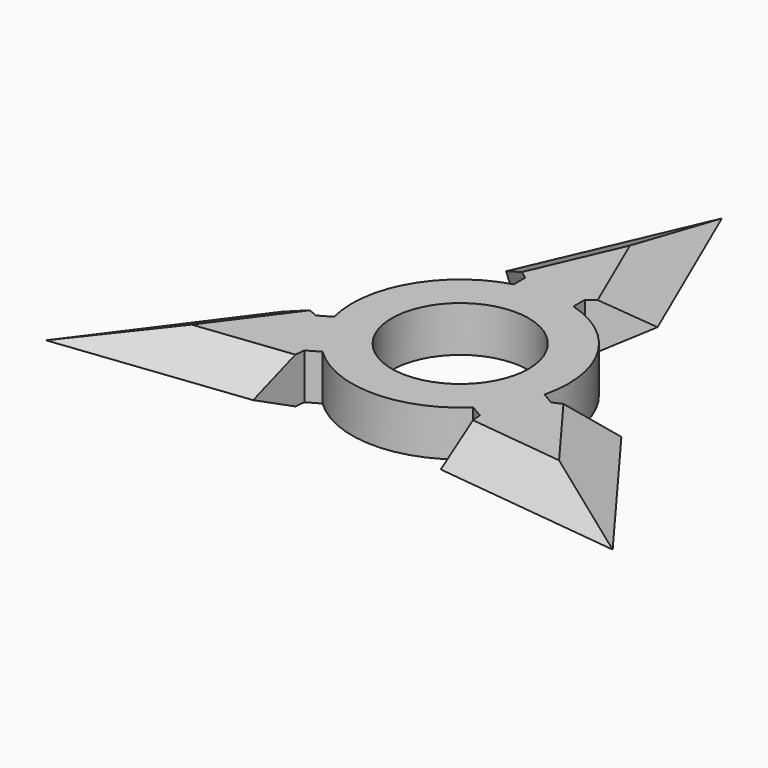
from build123d import *

# Parameters (mm, degrees)
F0_R            = 15.08125
F0_R_2          = 9.525
F1_DEPTH        = 6.35
F3_DEPTH        = 6.35
F3_COPIES_COUNT = 3
F4_SIZE2        = 3.175
F4_SIZE         = 6.35
F4_2_SIZE2      = 3.17499
F4_2_SIZE       = 6.34999


# Not quite as in the source:
# - a fillet or chamfer is up to 0.001 mm smaller than in the source, because OpenCascade refuses the exact size
# - a pattern or mirror of a feature is missing from the dataset's text; its kind, count and spacing are read off the source's solid


with BuildPart() as f1:
    # F0 (on Top) → F1 (new body)
    with BuildSketch(Plane.XY):
        Circle(F0_R)
        Circle(F0_R_2, mode=Mode.SUBTRACT)
    extrude(amount=F1_DEPTH)

    # F2 (on Top) → F3 (join, through all)
    with BuildSketch(Plane.XY):
        with BuildLine():
            Line((10.532929562, 21.1518518627), (0, 45.5084554851))
            Line((0, 45.5084554851), (-10.532929562, 21.1518518627))
            Line((-10.532929562, 21.1518518627), (-4.1548195295, 16.4949237317))
            Line((-4.1548195295, 16.4949237317), (-4.1548195295, 14.497640368))
            ThreePointArc((-4.1548195295, 14.497640368), (0, 15.08125), (4.1548195295, 14.497640368))
            Line((4.1548195295, 14.497640368), (4.1548195295, 16.4949237317))
            Line((4.1548195295, 16.4949237317), (10.532929562, 21.1518518627))
        make_face()
    f3 = extrude(amount=F3_DEPTH)

    # F3_copies: F3 ×3 about axis
    f3_copies_axis = Axis((0, 0, 0), (0, 0, 1))
    for i in range(1, F3_COPIES_COUNT):
        add(f3.rotate(f3_copies_axis, i * 360 / F3_COPIES_COUNT))

    # F4
    f4_edges = [f1.edges().sort_by_distance(p)[0] for p in [
        (-5.266465, 33.330154, 0),
        (5.266465, 33.330154, 0),
        (-31.497992, -12.104185, 0),
        (-26.231527, -21.225969, 0),
        (26.231527, -21.225969, 0),
        (31.497992, -12.104185, 0),
    ]]
    f4_side = f1.faces().sort_by_distance((3.11209, 15.496282, 0))[0]
    chamfer(f4_edges, length=F4_SIZE, length2=F4_SIZE2, reference=f4_side)

    # F4#2 (size 6.35 and 3.175 in the source; OpenCascade refuses exactly that, so slightly less here)
    f4_2_edges = [f1.edges().sort_by_distance(p)[0] for p in [
        (-5.266465, 33.330154, 6.35),
        (5.266465, 33.330154, 6.35),
        (-31.497992, -12.104185, 6.35),
        (-26.231527, -21.225969, 6.35),
        (26.231527, -21.225969, 6.35),
        (31.497992, -12.104185, 6.35),
    ]]
    f4_2_side = f1.faces().sort_by_distance((12.157715, 7.01926, 6.35))[0]
    chamfer(f4_2_edges, length=F4_2_SIZE, length2=F4_2_SIZE2, reference=f4_2_side)


solid = f1.part
